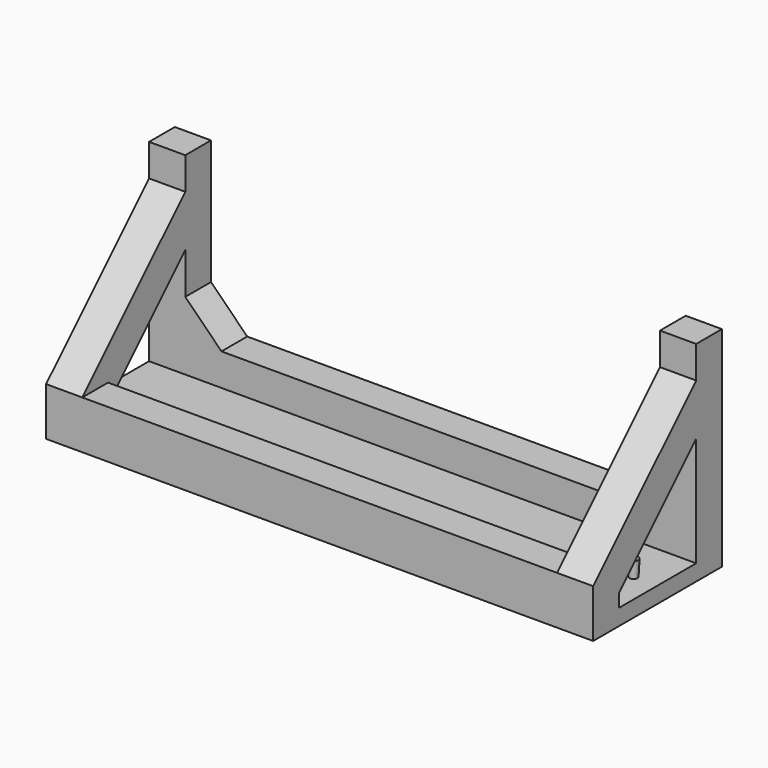
from build123d import *

# Parameters (mm, degrees)
F0_W      = 200
F0_H      = 20
F1_DEPTH  = 340
F2_W      = 40
F2_H      = 40
F3_DEPTH  = 340
F4_W      = 45
F4_H      = 40
F5_DEPTH  = 200
F7_DEPTH  = 45
F9_DEPTH  = 40
F10_R     = 5
F11_DEPTH = 20
F11_TAPER = -3


# Not quite as in the source:
# - a pattern or mirror of a feature is missing from the dataset's text; its kind, count and spacing are read off the source's solid


with BuildPart() as f1:
    # F0 (on Right) → F1 (new body, symmetric)
    with BuildSketch(Plane.YZ):
        Rectangle(F0_W, F0_H)
    extrude(amount=F1_DEPTH, both=True)

    # F2 (on Right) → F3 (join, symmetric)
    with BuildSketch(Plane.YZ):
        with Locations((80, 30)):
            Rectangle(F2_W, F2_H)
        with Locations((-80, 30)):
            Rectangle(F2_W, F2_H)
    extrude(amount=F3_DEPTH, both=True)

    # F4 (on face) → F5 (join)
    with BuildSketch(Plane.XY.offset(50)):
        with Locations((-317.5, 80)):
            Rectangle(F4_W, F4_H)
        with Locations((317.5, 80)):
            Rectangle(F4_W, F4_H)
    extrude(amount=F5_DEPTH)

    # F6 (on face) → F7 (join)
    with BuildSketch(Plane.YZ.offset(340)):
        Polygon((60, 210), (-100, 50), (-60, 50), (-60, 26.3603896932), (60, 146.3603896932), align=None)
    f7 = extrude(amount=-F7_DEPTH)

    # F7_copies: F7 across plane
    add(f7.mirror(Plane(origin=(0, 0, 0), x_dir=(0, 0, -1), z_dir=(-1, 0, 0))))

    # F8 (on face) → F9 (join)
    with BuildSketch(Plane(origin=(0, 100, 0), x_dir=(-1, 0, 0), z_dir=(0, 1, 0))):
        Polygon((-250, 50), (-295, 95), (-295, 50), align=None)
        Polygon((295, 50), (295, 95), (250, 50), align=None)
    extrude(amount=-F9_DEPTH)

    # F10 (on face) → F11 (join)
    with BuildSketch(Plane.XY.offset(10)):
        with Locations((310, 0)):
            Circle(F10_R)
    extrude(amount=F11_DEPTH, taper=F11_TAPER)


solid = f1.part
